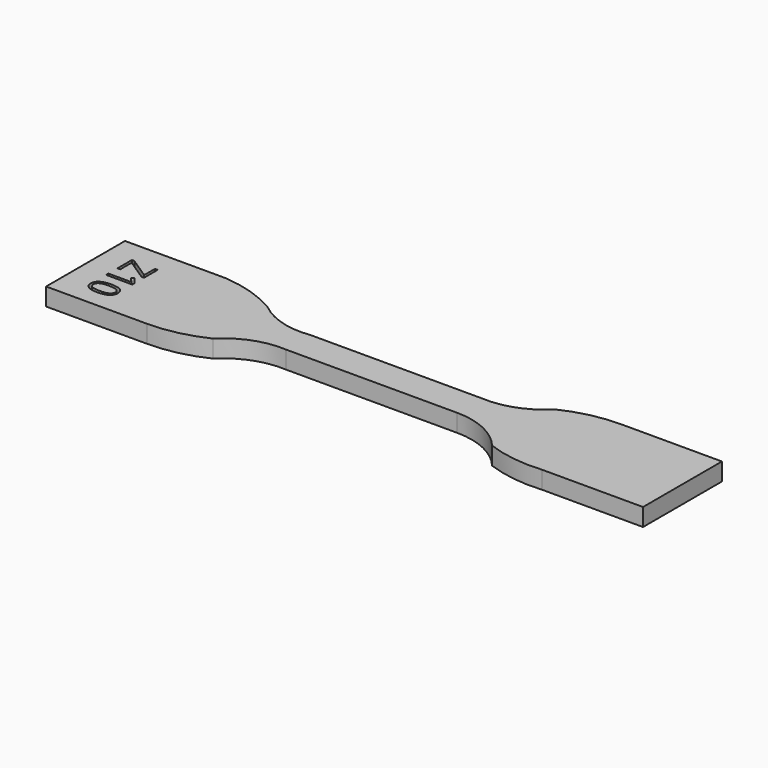
from build123d import *

# Parameters (mm, degrees)
F1_DEPTH     = 3.4
F2_TEXT_SIZE = 7.0564552314
F3_DEPTH     = 1


# Not quite as in the source:
# - Text() gives the source's letters only with a copy of the font that has no kerning and outlines rounded to 1/6400 em; it was checked with that copy


with BuildPart() as f1:
    # F0 (on Top) → F1 (new body)
    with BuildSketch(Plane.XY):
        with BuildLine():
            Line((-14.4320548165, 19.7811394548), (-33.8720548165, 19.7811394548))
            Line((-33.8720548165, 19.7811394548), (-33.8720548165, 0.7811394548))
            Line((-33.8720548165, 0.7811394548), (-14.4320548165, 0.7811394548))
            ThreePointArc((-14.4320548165, 0.7811394548), (-8.9053122052, 1.3996892086), (-3.6520548165, 3.2247301661))
            ThreePointArc((-3.6520548165, 3.2247301661), (1.3014698263, 6.4128780055), (7.1279451835, 7.2811394548))
            Line((7.1279451835, 7.2811394548), (40.1279451835, 7.2811394548))
            ThreePointArc((40.1279451835, 7.2811394548), (46.0837574042, 5.9511158081), (50.9079451835, 2.2137538538))
            ThreePointArc((50.9079451835, 2.2137538538), (56.2191047011, 0.9041953221), (61.6879451835, 0.7811394548))
            Line((61.6879451835, 0.7811394548), (81.1279451835, 0.7811394548))
            Line((81.1279451835, 0.7811394548), (81.1279451835, 19.7811394548))
            Line((81.1279451835, 19.7811394548), (61.6879451835, 19.7811394548))
            ThreePointArc((61.6879451835, 19.7811394548), (56.1612025723, 19.162589701), (50.9079451835, 17.3375487435))
            ThreePointArc((50.9079451835, 17.3375487435), (45.9544205407, 14.1494009041), (40.1279451835, 13.2811394548))
            Line((40.1279451835, 13.2811394548), (7.1279451835, 13.2811394548))
            ThreePointArc((7.1279451835, 13.2811394548), (1.4167452884, 13.6925537245), (-3.6520548165, 16.3560723447))
            ThreePointArc((-3.6520548165, 16.3560723447), (-8.8458057958, 18.686276846), (-14.4320548165, 19.7811394548))
        make_face()
    extrude(amount=F1_DEPTH)

    # F2 (on face) → F3 (cut)
    with BuildSketch(Plane.XY.offset(3.4)):
        with Locations(Location((-29.1824135929, 15.8650862949), (0, 0, -90))):
            Text('Z10', F2_TEXT_SIZE, font='Open Sans', text_align=(TextAlign.LEFT, TextAlign.BOTTOM))
    extrude(amount=-F3_DEPTH, mode=Mode.SUBTRACT)


solid = f1.part
